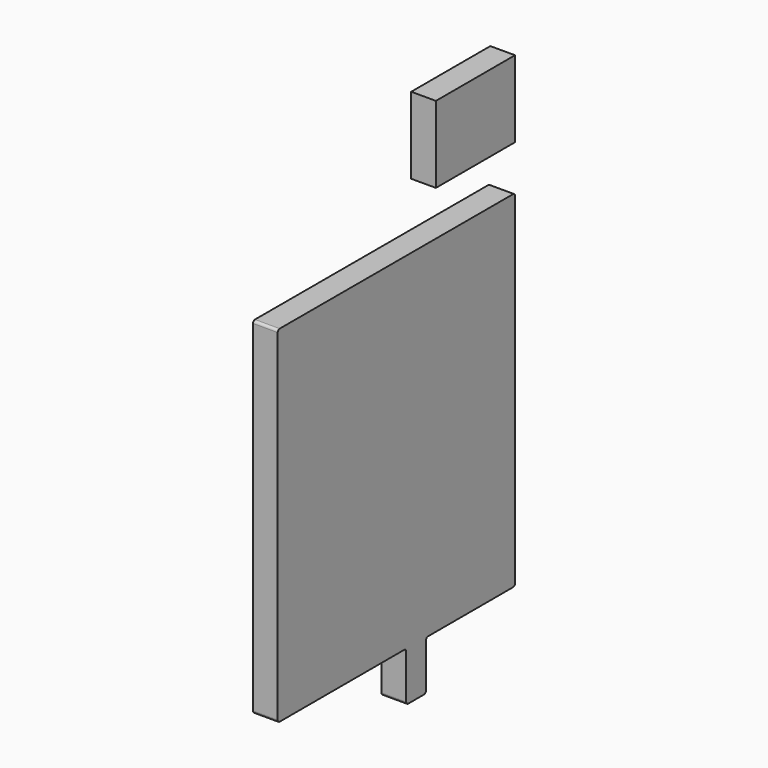
from build123d import *

# Parameters (mm, degrees)
F1_DEPTH = 5
F2_R     = 0.5
F3_R     = 0.5
F4_R     = 0.5


# Not quite as in the source:
# - a feature names something its author has since deleted; it is built from what else it names


with BuildPart() as f1:
    # F0 (on Right) → F1 (new body)
    with BuildSketch(Plane.YZ):
        Polygon((60, -0.0434386059), (0, 0), (0, -70), (12, -70), (12.4011761725, -70), (32.5, -70), (32.5, -80), (37.5, -80), (37.5, -70.0434386059), (60, -70.0434386059), align=None)
    extrude(amount=F1_DEPTH)

    # F2
    f2_edges = [f1.edges().sort_by_distance(p)[0] for p in [
        (2.5, 0, 0),
        (2.5, 0, -70),
        (2.5, 60, -70.043439),
        (2.5, 60, -0.043439),
    ]]
    fillet(f2_edges, radius=F2_R)

    # F3
    f3_edges = [f1.edges().sort_by_distance(p)[0] for p in [
        (2.5, 37.5, -70.043439),
        (2.5, 32.5, -70),
    ]]
    fillet(f3_edges, radius=F3_R)

    # F4
    f4_edges = [f1.edges().sort_by_distance(p)[0] for p in [
        (2.5, 32.5, -80),
        (2.5, 37.5, -80),
    ]]
    fillet(f4_edges, radius=F4_R)


with BuildPart() as f1b:
    # F0 (on Right) → F1, piece 2 (new body)
    with BuildSketch(Plane.YZ):
        Polygon((40, 8.9999613941), (42.5, 8.9999613941), (60, 8.9999613941), (60, 24.499980697), (42.5, 24.499980697), (40, 24.499980697), align=None)
    extrude(amount=F1_DEPTH)


solid = Compound([f1.part, f1b.part])
